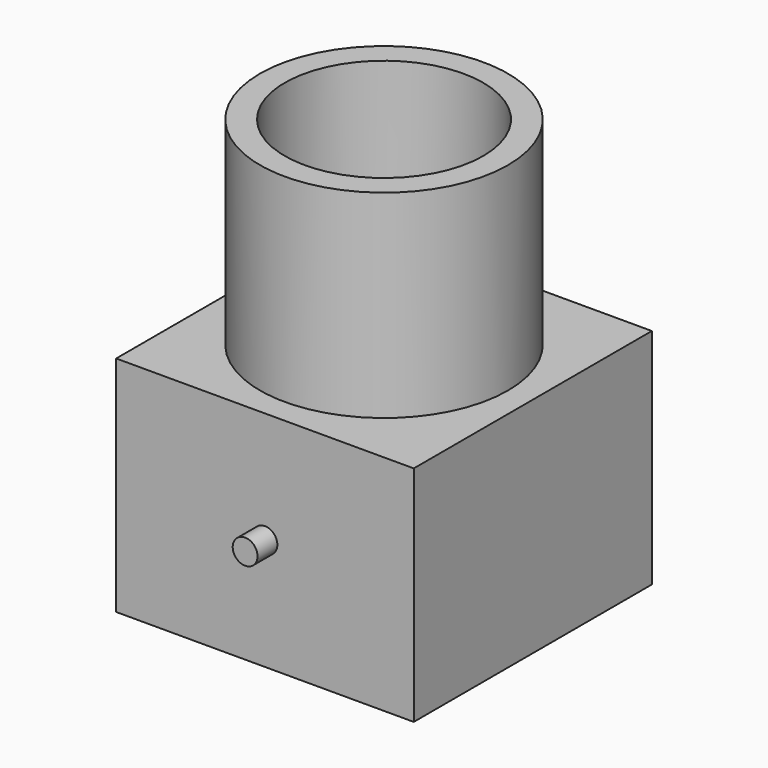
from build123d import *

# Parameters (mm, degrees)
F0_W          = 120
F0_H          = 120
F1_DEPTH      = 80
F2_T          = -10
F3_R          = 5
F4_DEPTH      = 70
F4_DEPTH_BACK = 55
F7_DEPTH      = 15
F9_DEPTH      = 5
F10_R         = 5
F11_DEPTH     = 5
F12_W         = 120
F12_H         = 120
F12_R         = 40
F13_DEPTH     = 10
F14_R         = 50
F14_R_2       = 40
F15_DEPTH     = 80


with BuildPart() as f1:
    # F0 (on Top) → F1 (new body)
    with BuildSketch(Plane.XY):
        Rectangle(F0_W, F0_H)
    extrude(amount=F1_DEPTH)

    # F2
    f2_openings = [f1.faces().sort_by_distance(p)[0] for p in [
        (0, 0, 80),
    ]]
    offset(amount=F2_T, openings=f2_openings)


with BuildPart() as f4:
    # F3 (on Front) → F4 (new body, two sides)
    with BuildSketch(Plane.XZ) as f4_sk:
        with Locations((0, 45)):
            Circle(F3_R)
    extrude(amount=F4_DEPTH)
    extrude(f4_sk.sketch, amount=-F4_DEPTH_BACK)


with BuildPart() as f1_1:
    add(f1.part)

    # F5: cut F4
    add(f4.part, mode=Mode.SUBTRACT)

    # F12 (on face) → F13 (join)
    with BuildSketch(Plane.XY.offset(80)):
        Rectangle(F12_W, F12_H)
        Circle(F12_R, mode=Mode.SUBTRACT)
    extrude(amount=F13_DEPTH)

    # F14 (on face) → F15 (join)
    with BuildSketch(Plane.XY.offset(90)):
        Circle(F14_R)
        Circle(F14_R_2, mode=Mode.SUBTRACT)
    extrude(amount=F15_DEPTH)


with BuildPart() as f4_1:
    add(f4.part)

    # F6 (on Front) → F7 (join, symmetric)
    with BuildSketch(Plane.XZ):
        with BuildLine():
            Line((-5.9844609002, 64.5206446149), (-28.2842712475, 35))
            ThreePointArc((-28.2842712475, 35), (0, 15), (28.2842712475, 35))
            Line((28.2842712475, 35), (5.9844609002, 64.5206446149))
            ThreePointArc((5.9844609002, 64.5206446149), (7.111028644, 62.3839613303), (7.5, 60))
            ThreePointArc((7.5, 60), (-2.3839613303, 52.888971356), (-5.9844609002, 64.5206446149))
        make_face()
        with BuildLine():
            ThreePointArc((5.9844609002, 64.5206446149), (0, 67.5), (-5.9844609002, 64.5206446149))
            ThreePointArc((-5.9844609002, 64.5206446149), (-2.3839613303, 52.888971356), (7.5, 60))
            ThreePointArc((7.5, 60), (7.111028644, 62.3839613303), (5.9844609002, 64.5206446149))
        make_face()
    extrude(amount=F7_DEPTH, both=True)

    # F8 (on Front) → F9 (cut, symmetric)
    with BuildSketch(Plane.XZ):
        with BuildLine():
            ThreePointArc((-28.2842712475, 35), (0, 15), (28.2842712475, 35))
            Line((28.2842712475, 35), (5.9844609002, 64.5206446149))
            ThreePointArc((5.9844609002, 64.5206446149), (0, 52.5), (-5.9844609002, 64.5206446149))
            Line((-5.9844609002, 64.5206446149), (-28.2842712475, 35))
        make_face()
    extrude(amount=F9_DEPTH, both=True, mode=Mode.SUBTRACT)


with BuildPart() as f11:
    # F10 (on Front) → F11 (new body, symmetric)
    with BuildSketch(Plane.XZ):
        with BuildLine():
            ThreePointArc((-17.3992636338, 61.875), (-0.9388520671, 42.5252022388), (17.5, 60))
            ThreePointArc((17.5, 60), (17.4747977612, 60.9388520671), (17.3992636338, 61.875))
            ThreePointArc((17.3992636338, 61.875), (0, 77.5), (-17.3992636338, 61.875))
        make_face()
        with BuildLine():
            ThreePointArc((-5.9844609002, 64.5206446149), (0, 67.5), (5.9844609002, 64.5206446149))
            ThreePointArc((5.9844609002, 64.5206446149), (0, 52.5), (-5.9844609002, 64.5206446149))
        make_face(mode=Mode.SUBTRACT)
        with BuildLine():
            ThreePointArc((-17.3992636338, 61.875), (0, 77.5), (17.3992636338, 61.875))
            Line((17.3992636338, 61.875), (9.9424363622, 131.0714285714))
            ThreePointArc((9.9424363622, 131.0714285714), (9.9855987207, 130.5364868955), (10, 130))
            ThreePointArc((10, 130), (-0.5364868955, 120.0144012793), (-9.9424363622, 131.0714285714))
            Line((-9.9424363622, 131.0714285714), (-17.3992636338, 61.875))
        make_face()
        with BuildLine():
            ThreePointArc((10, 130), (9.9855987207, 130.5364868955), (9.9424363622, 131.0714285714))
            ThreePointArc((9.9424363622, 131.0714285714), (0, 140), (-9.9424363622, 131.0714285714))
            ThreePointArc((-9.9424363622, 131.0714285714), (-0.5364868955, 120.0144012793), (10, 130))
        make_face()
        with Locations((0, 130)):
            Circle(F10_R, mode=Mode.SUBTRACT)
    extrude(amount=F11_DEPTH, both=True)


solid = Compound([f1_1.part, f4_1.part, f11.part])
